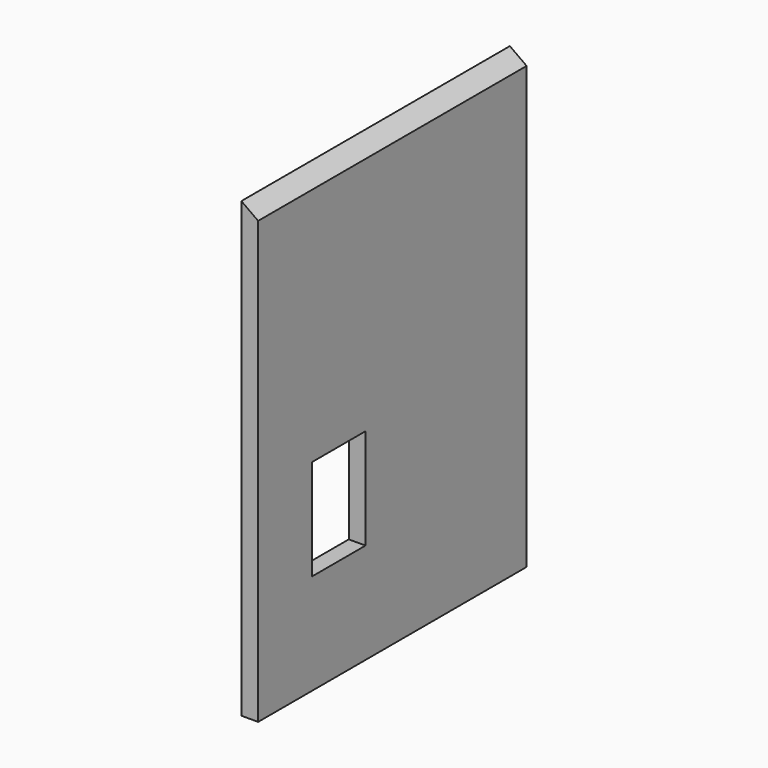
from build123d import *

# Parameters (mm, degrees)
F0_W     = 100
F0_H     = 80
F0_W_2   = 20
F0_H_2   = 30
F0_H_3   = 50
F0_H_4   = 5
F1_DEPTH = 2.5
F2_SIZE2 = 3.570407
F2_SIZE  = 4.99999


# Not quite as in the source:
# - a fillet or chamfer is up to 0.001 mm smaller than in the source, because OpenCascade refuses the exact size


with BuildPart() as f1:
    # F0 (on Right) → F1 (new body, symmetric)
    with BuildSketch(Plane.YZ):
        with Locations((-50, 40)):
            Rectangle(F0_W, F0_H)
        with Locations((-70, 40)):
            Rectangle(F0_W_2, F0_H_2, mode=Mode.SUBTRACT)
        with Locations((-50, 105)):
            Rectangle(F0_W, F0_H_3)
        with Locations((-50, -2.5)):
            Rectangle(F0_W, F0_H_4)
    extrude(amount=F1_DEPTH, both=True)

    # F2 (size 5 and 3.5704168108 in the source; OpenCascade refuses exactly that, so slightly less here)
    f2_edges = [f1.edges().sort_by_distance(p)[0] for p in [
        (2.5, -50, 130),
    ]]
    f2_side = f1.faces().sort_by_distance((0, -50, 130))[0]
    chamfer(f2_edges, length=F2_SIZE, length2=F2_SIZE2, reference=f2_side)


solid = f1.part
